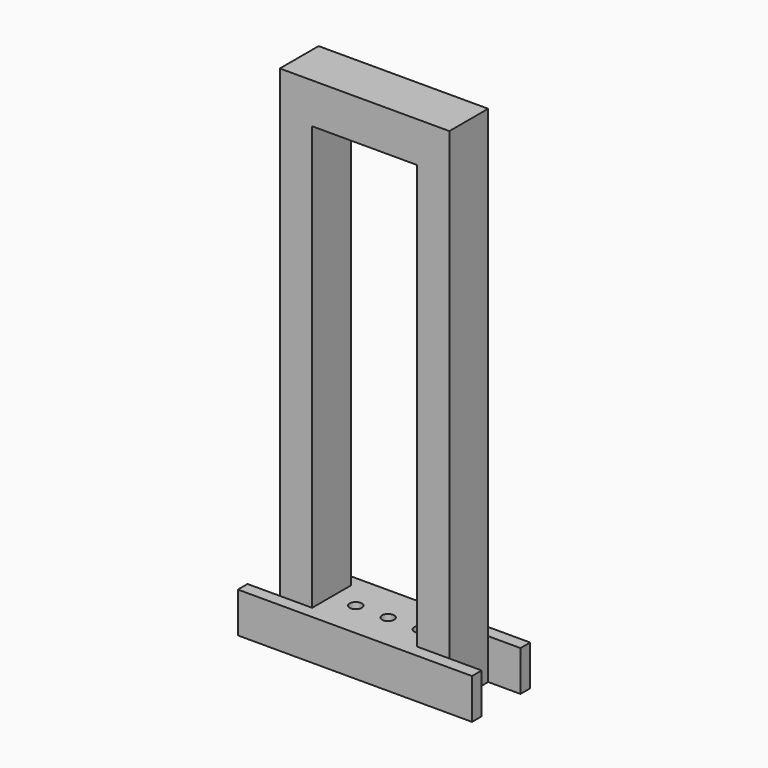
from build123d import *

# Parameters (mm, degrees)
F0_W     = 42
F0_H     = 12
F1_DEPTH = 10
F2_W     = 8
F2_H     = 12
F3_DEPTH = 105
F4_W     = 42
F4_H     = 12
F5_DEPTH = 10
F6_W     = 58
F6_H     = 10
F7_DEPTH = 3
F8_R     = 1.5
F9_DEPTH = 9.9999997765


# Not quite as in the source:
# - a pattern or mirror of a feature is missing from the dataset's text; its kind, count and spacing are read off the source's solid


with BuildPart() as f1:
    # F0 (on Top) → F1 (new body)
    with BuildSketch(Plane.XY):
        Rectangle(F0_W, F0_H)
    extrude(amount=F1_DEPTH)

    # F2 (on face) → F3 (join)
    with BuildSketch(Plane.XY.offset(10)):
        with Locations((-17, 0)):
            Rectangle(F2_W, F2_H)
        with Locations((17, 0)):
            Rectangle(F2_W, F2_H)
    extrude(amount=F3_DEPTH)

    # F4 (on face) → F5 (join)
    with BuildSketch(Plane.XY.offset(115)):
        Rectangle(F4_W, F4_H)
    extrude(amount=F5_DEPTH)

    # F6 (on face) → F7 (join)
    with BuildSketch(Plane.XZ.offset(6)):
        with Locations((0, 5)):
            Rectangle(F6_W, F6_H)
    f7 = extrude(amount=F7_DEPTH)

    # F7_copies: F7 across plane
    add(f7.mirror(Plane.ZX))

    # F8 (on face) → F9 (cut)
    with BuildSketch(Plane.XY.offset(10)):
        with Locations((-7, 0)):
            Circle(F8_R)
        with Locations((1, 0)):
            Circle(F8_R)
        with Locations((9, 0)):
            Circle(F8_R)
    extrude(amount=-F9_DEPTH, mode=Mode.SUBTRACT)


solid = f1.part
